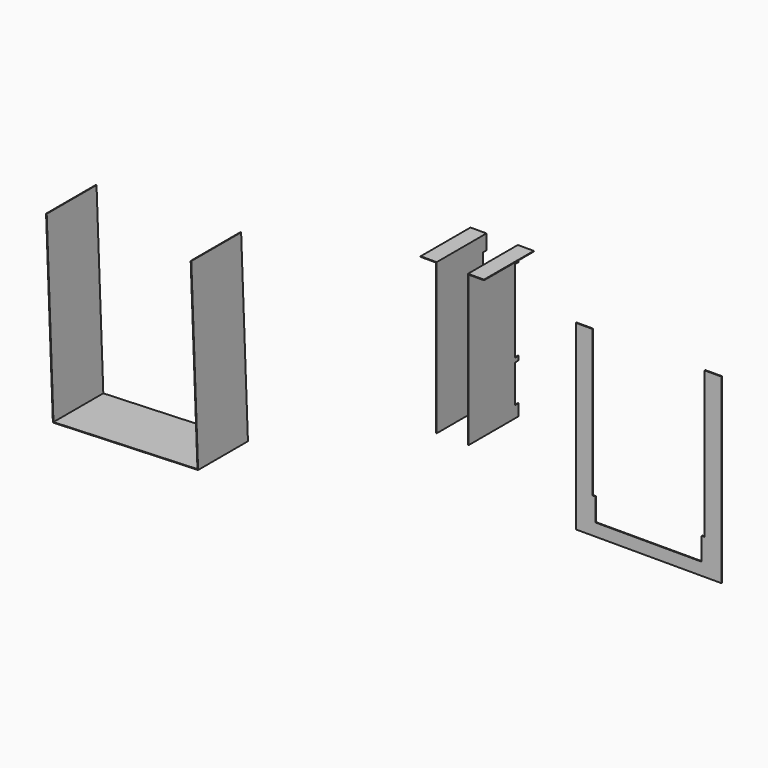
from build123d import *

# Parameters (mm, degrees)
F1_DEPTH  = 150
F3_DEPTH  = 150
F4_W      = 11
F4_H      = 198.4736350504
F4_H_2    = 90.5263649496
F5_DEPTH  = 1.5
F6_ANGLE  = 90
F10_DEPTH = 2


with BuildPart() as f1:
    # F0 (on Front) → F1 (new body)
    with BuildSketch(Plane.XZ):
        Polygon((-291.8999160505, -297.8952373376), (-308.294596378, 139.7978223024), (-309.7935452124, 139.7416761369), (-293.4550110503, -296.4524346687), (-640.2118414044, -309.4409142889), (-656.5503755664, 126.7531965167), (-658.0493244007, 126.6970503512), (-641.6546440732, -310.9960092888), align=None)
    extrude(amount=F1_DEPTH)


with BuildPart() as f3:
    # F2 (on Right) → F3 (new body)
    with BuildSketch(Plane.YZ):
        Polygon((148.654194653, 154.7818724839), (148.654194653, 156.2818724839), (110.154194653, 156.2818724839), (110.154194653, -206.7181275161), (111.654194653, -206.7181275161), (111.654194653, 154.7818724839), align=None)
    extrude(amount=F3_DEPTH)

    # F4 (on face) → F5 (cut)
    with BuildSketch(Plane(origin=(0, 111.654194653, 0), x_dir=(-1, 0, 0), z_dir=(0, 1, 0))):
        with Locations((-5.5, 21.0450549587)):
            Rectangle(F4_W, F4_H)
        with Locations((-5.5, -133.4549450413)):
            Rectangle(F4_W, F4_H_2)
    extrude(amount=-F5_DEPTH, mode=Mode.SUBTRACT)


with BuildPart() as f3_1:
    # F6: moved
    add(f3.part.rotate(Axis((150, 110.154194653, -25.2181275161), (0, 0, -1)), F6_ANGLE))


with BuildPart() as f7_1:
    # F7: copy of F3
    add(f3_1.part.moved(Location((-37, 0, 0))))


with BuildPart() as f7_1_1:
    # F8: moved
    add(f7_1.part.moved(Location((-38.5, 0, 0))))


with BuildPart() as f10:
    # F9 (on Front) → F10 (new body)
    with BuildSketch(Plane.XZ):
        Polygon((849.6708440304, -226.6395755177), (849.6708440304, 211.3604244823), (809.6708440304, 211.3604244823), (809.6708440304, -141.6395755177), (802.6708440304, -141.6395755177), (802.6708440304, -196.6395755177), (546.6708440304, -196.6395755177), (546.6708440304, -141.6395755177), (539.6708440304, -141.6395755177), (539.6708440304, 211.3604244823), (499.6708440304, 211.3604244823), (499.6708440304, -226.6395755177), align=None)
    extrude(amount=F10_DEPTH)


with BuildPart() as f11_1:
    # F11: instance of F7_1
    add(f7_1_1.part.mirror(Plane(origin=(74.5, 180.8449262557, -25.0859104705), x_dir=(0, -1, 0), z_dir=(-1, 0, 0))))


solid = Compound([f1.part, f3_1.part, f10.part, f11_1.part])
